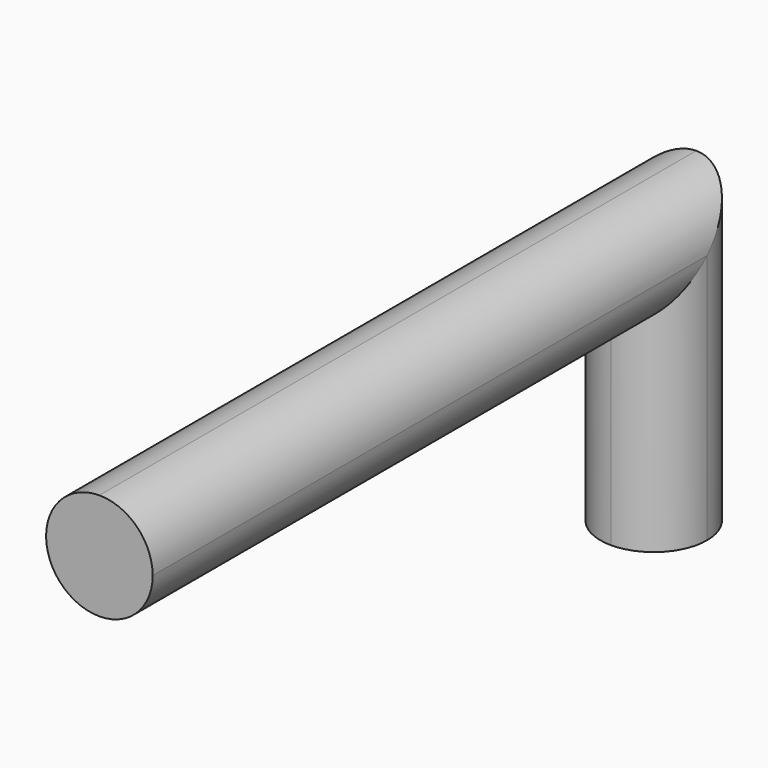
from build123d import *

# Parameters (mm, degrees)
F1_DEPTH = 10
F2_R     = 4.99999


# Not quite as in the source:
# - a fillet or chamfer is up to 0.001 mm smaller than in the source, because OpenCascade refuses the exact size


with BuildPart() as f1:
    # F0 (on Right) → F1 (new body)
    with BuildSketch(Plane.YZ):
        Polygon((0, 18.5156259346), (0, 0), (10, 0), (10, 28.5156259346), (-60, 28.5156259346), (-60, 18.5156259346), align=None)
    extrude(amount=F1_DEPTH)

    # F2 (radius 5 in the source; OpenCascade refuses exactly that, so slightly less here)
    f2_edges = [f1.edges().sort_by_distance(p)[0] for p in [
        (10, -30, 18.515626),
        (0, -30, 18.515626),
        (10, -25, 28.515626),
        (0, -25, 28.515626),
        (10, 0, 9.257813),
        (0, 0, 9.257813),
        (0, 10, 14.257813),
        (10, 10, 14.257813),
    ]]
    fillet(f2_edges, radius=F2_R)


solid = f1.part
